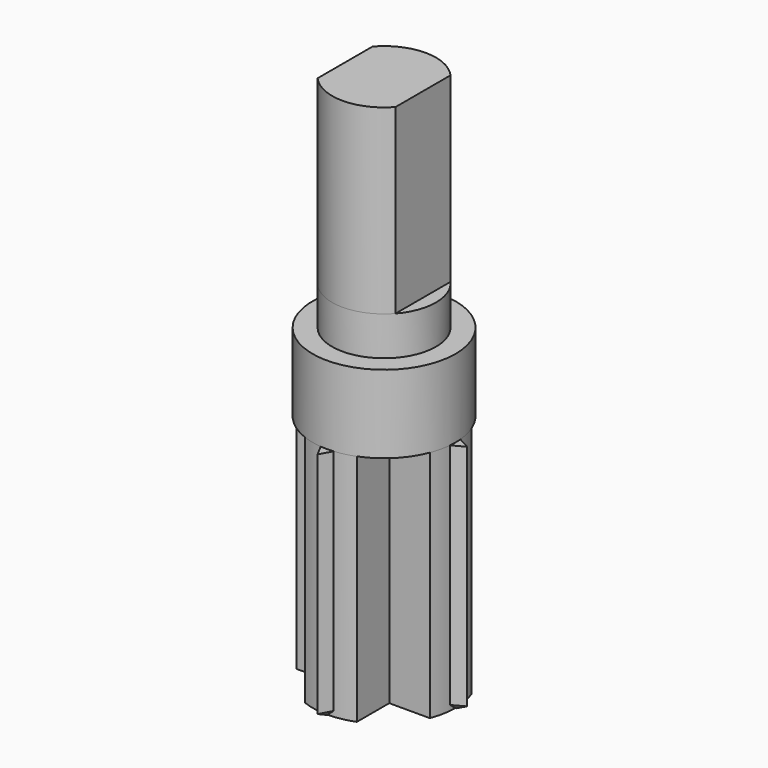
from build123d import *

# Parameters (mm, degrees)
F0_R     = 2.75
F0_R_2   = 2
F1_DEPTH = 3
F2_DEPTH = 1.5
F4_DEPTH = 7
F6_DEPTH = 9
F7_SIZE  = 0.2


# Not quite as in the source:
# - after a boolean that leaves OpenCascade's solid faulty, fix() repairs it


with BuildPart() as f1:
    # F0 (on Top) → F1 (new body)
    with BuildSketch(Plane.XY):
        Circle(F0_R)
        Circle(F0_R_2, mode=Mode.SUBTRACT)
        Circle(F0_R_2)
    extrude(amount=-F1_DEPTH)

    # F0 (on Top) → F2 (join)
    with BuildSketch(Plane.XY):
        Circle(F0_R_2)
    extrude(amount=F2_DEPTH)

    # F3 (on face) → F4 (join)
    with BuildSketch(Plane.XY.offset(1.5)):
        with BuildLine():
            ThreePointArc((1.5, 1.3228756555), (0, 2), (-1.5, 1.3228756555))
            Line((-1.5, 1.3228756555), (-1.5, -1.3228756555))
            ThreePointArc((-1.5, -1.3228756555), (0, -2), (1.5, -1.3228756555))
            Line((1.5, -1.3228756555), (1.5, 1.3228756555))
        make_face()
    extrude(amount=F4_DEPTH)

    # F5 (on face) → F6 (join)
    with BuildSketch(Plane(origin=(0, 0, -3), x_dir=(1, 0, 0), z_dir=(0, 0, -1))):
        with BuildLine():
            ThreePointArc((0.25, -2.7386127875), (0.63122595, -2.676575013), (1, -2.5617376915))
            Line((1, -2.5617376915), (1, -1))
            Line((1, -1), (2.5617376915, -1))
            ThreePointArc((2.5617376915, -1), (2.676575013, -0.63122595), (2.7386127875, -0.25))
            ThreePointArc((2.7386127875, -0.25), (2.7471517218, -0.1251296014), (2.75, 0))
            ThreePointArc((2.75, 0), (2.7471517218, 0.1251296014), (2.7386127875, 0.25))
            ThreePointArc((2.7386127875, 0.25), (2.676575013, 0.63122595), (2.5617376915, 1))
            Line((2.5617376915, 1), (1, 1))
            Line((1, 1), (1, 2.5617376915))
            ThreePointArc((1, 2.5617376915), (0.63122595, 2.676575013), (0.25, 2.7386127875))
            ThreePointArc((0.25, 2.7386127875), (0, 2.75), (-0.25, 2.7386127875))
            ThreePointArc((-0.25, 2.7386127875), (-0.63122595, 2.676575013), (-1, 2.5617376915))
            Line((-1, 2.5617376915), (-1, 1))
            Line((-1, 1), (-2.5617376915, 1))
            ThreePointArc((-2.5617376915, 1), (-2.676575013, 0.63122595), (-2.7386127875, 0.25))
            ThreePointArc((-2.7386127875, 0.25), (-2.75, 0), (-2.7386127875, -0.25))
            ThreePointArc((-2.7386127875, -0.25), (-2.676575013, -0.63122595), (-2.5617376915, -1))
            Line((-2.5617376915, -1), (-1, -1))
            Line((-1, -1), (-1, -2.5617376915))
            ThreePointArc((-1, -2.5617376915), (-0.63122595, -2.676575013), (-0.25, -2.7386127875))
            ThreePointArc((-0.25, -2.7386127875), (0, -2.75), (0.25, -2.7386127875))
        make_face()
        with BuildLine():
            ThreePointArc((2.75, 0), (2.7471517218, -0.1251296014), (2.7386127875, -0.25))
            Line((2.7386127875, -0.25), (3.2, 0))
            Line((3.2, 0), (2.7386127875, 0.25))
            ThreePointArc((2.7386127875, 0.25), (2.7471517218, 0.1251296014), (2.75, 0))
        make_face()
        with BuildLine():
            Line((0, -3.2), (0.25, -2.7386127875))
            ThreePointArc((0.25, -2.7386127875), (0, -2.75), (-0.25, -2.7386127875))
            Line((-0.25, -2.7386127875), (0, -3.2))
        make_face()
        with BuildLine():
            Line((-3.2, 0), (-2.7386127875, -0.25))
            ThreePointArc((-2.7386127875, -0.25), (-2.75, 0), (-2.7386127875, 0.25))
            Line((-2.7386127875, 0.25), (-3.2, 0))
        make_face()
        with BuildLine():
            ThreePointArc((-0.25, 2.7386127875), (0, 2.75), (0.25, 2.7386127875))
            Line((0.25, 2.7386127875), (0, 3.2))
            Line((0, 3.2), (-0.25, 2.7386127875))
        make_face()
    extrude(amount=F6_DEPTH)

    add(f1.part.fix(), mode=Mode.REPLACE)

    # F7
    f7_edges = [f1.edges().sort_by_distance(p)[0] for p in [
        (-0.125, 2.969306, -12),
        (0.125, 2.969306, -12),
        (-2.969306, 0.125, -12),
        (-2.969306, -0.125, -12),
        (0.125, -2.969306, -12),
        (-0.125, -2.969306, -12),
        (2.969306, -0.125, -12),
        (2.969306, 0.125, -12),
    ]]
    chamfer(f7_edges, length=F7_SIZE)


solid = f1.part
